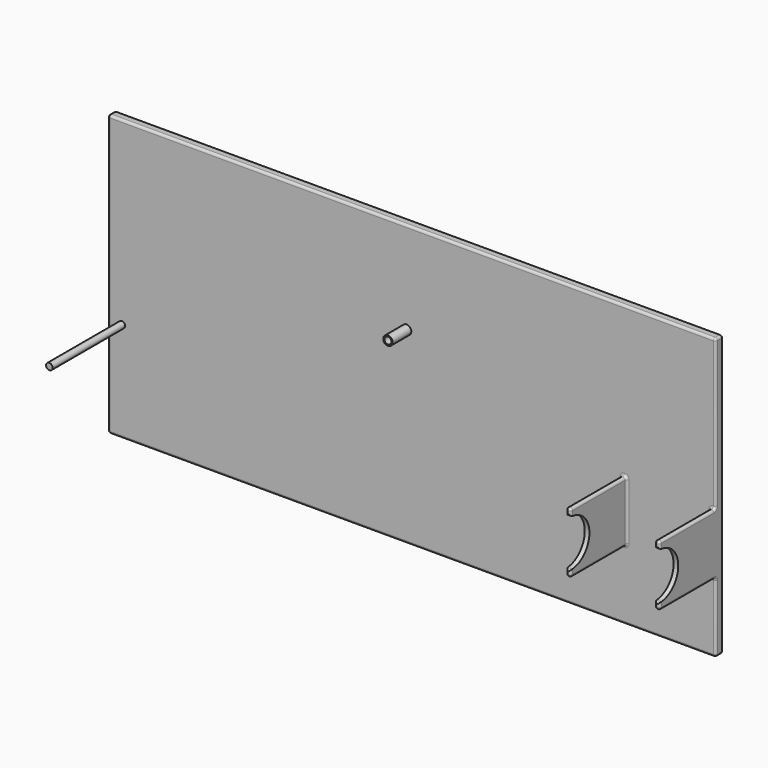
from build123d import *

# Parameters (mm, degrees)
F0_W      = 1300
F0_H      = 214.1299426556
F0_H_2    = 385.8700573444
F1_DEPTH  = 20
F2_W      = 5
F2_H      = 130
F3_DEPTH  = 150
F4_R      = 50
F5_DEPTH  = 2015
F6_R      = 4.99999
F7_R      = 7.5
F8_DEPTH  = 20.001
F7_R_2    = 10
F9_DEPTH  = 50
F10_R     = 7
F11_DEPTH = 194


# Not quite as in the source:
# - a fillet or chamfer is up to 0.001 mm smaller than in the source, because OpenCascade refuses the exact size


with BuildPart() as f1:
    # F0 (on Front) → F1 (new body)
    with BuildSketch(Plane.XZ):
        with Locations((309.8854213953, -107.0649713278)):
            Rectangle(F0_W, F0_H)
        with Locations((309.8854213953, 192.9350286722)):
            Rectangle(F0_W, F0_H_2)
    extrude(amount=F1_DEPTH)

    # F2 (on face) → F3 (join)
    with BuildSketch(Plane.XZ.offset(20)):
        Polygon((949.8854213953, 65), (949.8854213953, 0), (949.8854213953, -65), (954.8854213953, -65), (954.8854213953, 65), align=None)
        with Locations((762.3854213953, 0)):
            Rectangle(F2_W, F2_H)
        Polygon((769.8854213953, 65), (764.8854213953, 65), (764.8854213953, -65), (769.8854213953, -65), (769.8854213953, 0), align=None)
        with Locations((957.3854213953, 0)):
            Rectangle(F2_W, F2_H)
    extrude(amount=F3_DEPTH)

    # F4 (on face) → F5 (cut)
    with BuildSketch(Plane.YZ.offset(959.8854213953)):
        with Locations((-170, 0)):
            Circle(F4_R)
    extrude(amount=-F5_DEPTH, mode=Mode.SUBTRACT)

    # F6 (radius 5 in the source; OpenCascade refuses exactly that, so slightly less here)
    f6_edges = [f1.edges().sort_by_distance(p)[0] for p in [
        (764.885421, -170, -50),
        (769.885421, -170, -57.5),
        (764.885421, -170, -65),
        (759.885421, -170, -57.5),
        (764.885421, -170, 65),
        (769.885421, -170, 57.5),
        (764.885421, -170, 50),
        (759.885421, -170, 57.5),
        (759.885421, -95, -65),
        (769.885421, -95, -65),
        (764.885421, -20, -65),
        (769.885421, -95, 65),
        (759.885421, -95, 65),
        (764.885421, -20, 65),
        (954.885421, -170, 65),
        (959.885421, -170, 57.5),
        (954.885421, -170, 50),
        (949.885421, -170, 57.5),
        (954.885421, -170, -50),
        (959.885421, -170, -57.5),
        (954.885421, -170, -65),
        (949.885421, -170, -57.5),
        (949.885421, -95, -65),
        (959.885421, -95, -65),
        (954.885421, -20, -65),
        (959.885421, -95, 65),
        (949.885421, -95, 65),
        (954.885421, -20, 65),
        (309.885421, 0, 385.870057),
        (959.885421, -10, 385.870057),
        (-340.114579, -10, 385.870057),
        (309.885421, -20, 385.870057),
        (-340.114579, -10, -214.129943),
        (959.885421, -10, -214.129943),
        (309.885421, 0, -214.129943),
        (309.885421, -20, -214.129943),
        (959.885421, 0, 85.870057),
        (-340.114579, 0, 85.870057),
        (-340.114579, -20, 85.870057),
        (959.885421, -20, 225.435029),
        (949.885421, -20, 0),
        (959.885421, -20, -139.564971),
        (759.885421, -20, 0),
        (769.885421, -20, 0),
    ]]
    fillet(f6_edges, radius=F6_R)

    # F7 (on face) → F8 (cut, through all)
    with BuildSketch(Plane.XZ.offset(20)):
        with Locations((298.8854213953, 188.5)):
            Circle(F7_R)
    extrude(amount=-F8_DEPTH, mode=Mode.SUBTRACT)

    # F7 (on face) → F9 (join)
    with BuildSketch(Plane.XZ.offset(20)):
        with Locations((298.8854213953, 188.5)):
            Circle(F7_R_2)
        with Locations((298.8854213953, 188.5)):
            Circle(F7_R, mode=Mode.SUBTRACT)
    extrude(amount=F9_DEPTH)

    # F10 (on face) → F11 (join)
    with BuildSketch(Plane.XZ.offset(20)):
        with Locations((-310.1145786047, 0)):
            Circle(F10_R)
    extrude(amount=F11_DEPTH)


solid = f1.part
